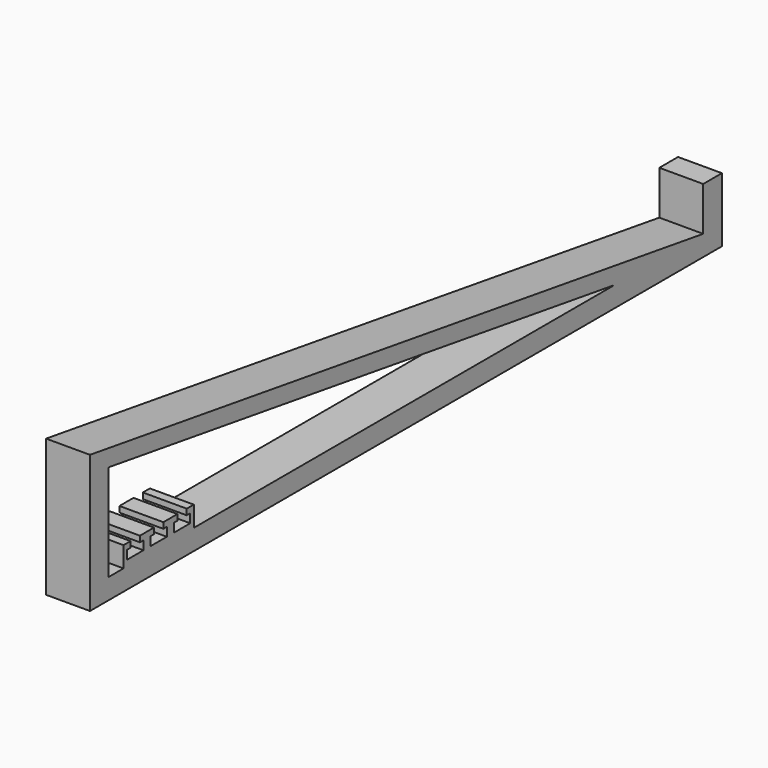
from build123d import *

# Parameters (mm, degrees)
F1_DEPTH = 15


# Not quite as in the source:
# - ends of sketch curves that miss each other by under 0.0002 mm in the source are joined


with BuildPart() as f1:
    # F0 (on Right) → F1 (new body)
    with BuildSketch(Plane.YZ):
        Polygon((86.4749986591, 7), (132.3186528001, 0), (132.3186528001, 22), (124.3186528001, 22), (124.3186528001, 7), align=None)
        Polygon((-129.6450851485, 0), (132.3186528001, 0), (86.4749986591, 7), (-93.3098772168, 7), (-103.3098761737, 7), (-113.3098740876, 7), (-123.3098730445, 7), (-129.6450851485, 7), align=None)
        Polygon((-129.6450851485, 40), (86.4749986591, 7), (124.3186528001, 7), (-137.6450851485, 47), (-137.6450851485, 0), (-129.6450851485, 0), (-129.6450851485, 7), align=None)
        Polygon((-123.3098730445, 14), (-123.3098730445, 7), (-113.3098740876, 7), (-113.3098730445, 14), (-116.3098730445, 14), (-116.3098730445, 12), (-114.8098730445, 12), (-114.8098730445, 9), (-121.8098730445, 9), (-121.8098730445, 12), (-120.3098730445, 12), (-120.3098730445, 14), align=None)
        Polygon((-113.3098740876, 7), (-103.3098761737, 7), (-103.3098751307, 14), (-106.3098751307, 14), (-106.3098751307, 12), (-104.8098751307, 12), (-104.8098751307, 9), (-111.8098751307, 9), (-111.8098751307, 12), (-110.3098751307, 12), (-110.3098751307, 14), (-113.3098751307, 14), align=None)
        Polygon((-103.3098761737, 7), (-93.3098772168, 7), (-93.3098772168, 14), (-96.3098772168, 14), (-96.3098772168, 12), (-94.8098772168, 12), (-94.8098772168, 9), (-101.8098772168, 9), (-101.8098772168, 12), (-100.3098772168, 12), (-100.3098772168, 14), (-103.3098772168, 14), align=None)
    extrude(amount=F1_DEPTH)


solid = f1.part
